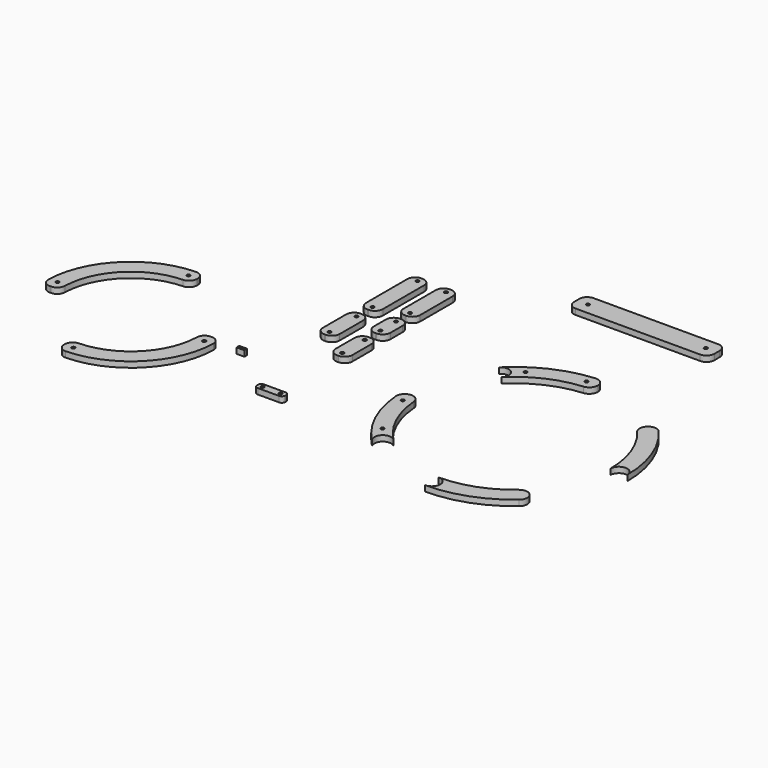
from build123d import *

# Parameters (mm, degrees)
F0_R     = 1.5
F1_DEPTH = 5.08
F0_W     = 7
F0_H     = 3
F0_W_2   = 5.08
F0_H_2   = 1.5
F0_W_3   = 12.5
F0_H_3   = 7
F0_W_4   = 15
F0_H_4   = 60
F0_H_5   = 40
F0_H_6   = 35
F0_H_7   = 27.5
F0_H_8   = 50
F0_W_5   = 125
F0_H_9   = 20
F2_R     = 7
F2_2_R   = 7
F2_3_R   = 7
F2_4_R   = 7
F2_5_R   = 7
F2_6_R   = 7
F2_7_R   = 7
F2_8_R   = 7
F3_R     = 3
F4_R     = 7.49999
F4_2_R   = 7.49999
F4_3_R   = 7.49999
F4_4_R   = 7.49999


# Not quite as in the source:
# - a fillet or chamfer is up to 0.001 mm smaller than in the source, because OpenCascade refuses the exact size
# - a feature names something its author has since deleted; it is built from what else it names


with BuildPart() as f1:
    # F0 (on Top) → F1 (new body)
    with BuildSketch(Plane.XY):
        with BuildLine():
            Line((-60.3335389302, 75.6855827492), (-60.3335389302, 90.7311393763))
            ThreePointArc((-60.3335389302, 90.7311393763), (-118.5826653378, 68.9457537369), (-140.3680509771, 10.6966273294))
            Line((-140.3680509771, 10.6966273294), (-125.32249435, 10.6966273294))
            ThreePointArc((-125.32249435, 10.6966273294), (-107.97606362, 58.3391520191), (-60.3335389302, 75.6855827492))
        make_face()
        with Locations((-133.0496567488, 18.6966273294)):
            Circle(F0_R, mode=Mode.SUBTRACT)
        with Locations((-68.3335389302, 83.4127451479)):
            Circle(F0_R, mode=Mode.SUBTRACT)
    extrude(amount=F1_DEPTH)

    # F2
    f2_edges = [f1.edges().sort_by_distance(p)[0] for p in [
        (-140.368051, 10.696627, 2.54),
        (-125.322494, 10.696627, 2.54),
        (-60.333539, 90.731139, 2.54),
        (-60.333539, 75.685583, 2.54),
    ]]
    fillet(f2_edges, radius=F2_R)


with BuildPart() as f1b:
    # F0 (on Top) → F1, piece 2 (new body)
    with BuildSketch(Plane.XY):
        with BuildLine():
            ThreePointArc((-70.7657745674, -58.9056490804), (-14.3940550828, -38.933443582), (9.4503432512, 15.9127451479))
            ThreePointArc((9.4503432512, 15.9127451479), (9.404928058, 18.5223842874), (9.2687374795, 21.1288629665))
            Line((9.2687374795, 21.1288629665), (-5.7768191475, 21.1288629665))
            ThreePointArc((-5.7768191475, 21.1288629665), (-5.6064742504, 18.5232761214), (-5.5496567488, 15.9127451479))
            ThreePointArc((-5.5496567488, 15.9127451479), (-25.0093500721, -28.3194098364), (-70.7657745674, -43.8600924533))
            Line((-70.7657745674, -43.8600924533), (-70.7657745674, -58.9056490804))
        make_face()
        with Locations((-62.7657745674, -51.5872548521)):
            Circle(F0_R, mode=Mode.SUBTRACT)
        with Locations((1.9503432512, 13.1288629665)):
            Circle(F0_R, mode=Mode.SUBTRACT)
    extrude(amount=F1_DEPTH)

    # F2#2
    f2_2_edges = [f1b.edges().sort_by_distance(p)[0] for p in [
        (-5.776819, 21.128863, 2.54),
        (9.268737, 21.128863, 2.54),
        (-70.765775, -43.860092, 2.54),
        (-70.765775, -58.905649, 2.54),
    ]]
    fillet(f2_2_edges, radius=F2_2_R)


with BuildPart() as f1c:
    # F0 (on Top) → F1, piece 3 (new body)
    with BuildSketch(Plane.XY):
        with Locations((29.0703890151, 21.1699748555)):
            Rectangle(F0_W, F0_H)
        with Locations((29.0703890151, 21.1699748555)):
            Rectangle(F0_W_2, F0_H_2, mode=Mode.SUBTRACT)
    extrude(amount=F1_DEPTH)


with BuildPart() as f1d:
    # F0 (on Top) → F1, piece 4 (new body)
    with BuildSketch(Plane.XY):
        with Locations((78.5480350256, -15.4045127481)):
            Rectangle(F0_W_3, F0_H_3)
        with Locations((76.7980350256, -15.4045127481)):
            Circle(F0_R, mode=Mode.SUBTRACT)
        with Locations((91.0480350256, -15.4045127481)):
            Rectangle(F0_W_3, F0_H_3)
        with Locations((92.7980350256, -15.4045127481)):
            Circle(F0_R, mode=Mode.SUBTRACT)
    extrude(amount=F1_DEPTH)

    # F3
    f3_edges = [f1d.edges().sort_by_distance(p)[0] for p in [
        (72.298035, -11.904513, 2.54),
        (72.298035, -18.904513, 2.54),
        (97.298035, -11.904513, 2.54),
        (97.298035, -18.904513, 2.54),
    ]]
    fillet(f3_edges, radius=F3_R)


with BuildPart() as f1e:
    # F0 (on Top) → F1, piece 5 (new body)
    with BuildSketch(Plane.XY):
        with BuildLine():
            Line((257.5643956661, 124.5856685936), (257.5643956661, 139.5856685936))
            ThreePointArc((257.5643956661, 139.5856685936), (219.2960524296, 131.9736218448), (186.8537175475, 110.2963467123))
            ThreePointArc((186.8537175475, 110.2963467123), (197.4603192653, 110.2963467123), (197.4603192653, 99.6897449945))
            ThreePointArc((197.4603192653, 99.6897449945), (225.0363039151, 118.1154288571), (257.5643956661, 124.5856685936))
        make_face()
        with Locations((205.6464472819, 116.1413779534)):
            Circle(F0_R, mode=Mode.SUBTRACT)
        with Locations((247.5643956661, 131.5435393824)):
            Circle(F0_R, mode=Mode.SUBTRACT)
    extrude(amount=F1_DEPTH)

    # F4 (radius 7.5 in the source; OpenCascade refuses exactly that, so slightly less here)
    f4_edges = [f1e.edges().sort_by_distance(p)[0] for p in [
        (257.564396, 139.585669, 2.54),
        (257.564396, 124.585669, 2.54),
    ]]
    fillet(f4_edges, radius=F4_R)


with BuildPart() as f1f:
    # F0 (on Top) → F1, piece 6 (new body)
    with BuildSketch(Plane.XY):
        with BuildLine():
            ThreePointArc((342.5643956661, 39.5856685936), (350.0643956661, 47.0856685936), (357.5643956661, 39.5856685936))
            ThreePointArc((357.5643956661, 39.5856685936), (349.9523489173, 77.8540118302), (328.2750737848, 110.2963467123))
            Line((328.2750737848, 110.2963467123), (317.668472067, 99.6897449945))
            ThreePointArc((317.668472067, 99.6897449945), (336.0941559296, 72.1137603447), (342.5643956661, 39.5856685936))
        make_face()
    extrude(amount=F1_DEPTH)

    # F4#2 (radius 7.5 in the source; OpenCascade refuses exactly that, so slightly less here)
    f4_2_edges = [f1f.edges().sort_by_distance(p)[0] for p in [
        (328.275074, 110.296347, 2.54),
        (317.668472, 99.689745, 2.54),
    ]]
    fillet(f4_2_edges, radius=F4_2_R)


with BuildPart() as f1g:
    # F0 (on Top) → F1, piece 7 (new body)
    with BuildSketch(Plane.XY):
        with BuildLine():
            ThreePointArc((157.5643956661, 39.5856685936), (165.176442415, 1.3173253571), (186.8537175475, -31.125009525))
            ThreePointArc((186.8537175475, -31.125009525), (186.8537175475, -20.5184078072), (197.4603192653, -20.5184078072))
            ThreePointArc((197.4603192653, -20.5184078072), (179.0346354027, 7.0575768426), (172.5643956661, 39.5856685936))
            Line((172.5643956661, 39.5856685936), (157.5643956661, 39.5856685936))
        make_face()
        with Locations((181.0086863064, -12.3322797906)):
            Circle(F0_R, mode=Mode.SUBTRACT)
        with Locations((165.6065248774, 29.5856685936)):
            Circle(F0_R, mode=Mode.SUBTRACT)
    extrude(amount=F1_DEPTH)

    # F4#4 (radius 7.5 in the source; OpenCascade refuses exactly that, so slightly less here)
    f4_4_edges = [f1g.edges().sort_by_distance(p)[0] for p in [
        (157.564396, 39.585669, 2.54),
        (172.564396, 39.585669, 2.54),
    ]]
    fillet(f4_4_edges, radius=F4_4_R)


with BuildPart() as f1h:
    # F0 (on Top) → F1, piece 8 (new body)
    with BuildSketch(Plane.XY):
        with BuildLine():
            ThreePointArc((257.5643956661, -60.4143314064), (295.8327389026, -52.8022846575), (328.2750737848, -31.125009525))
            Line((328.2750737848, -31.125009525), (317.668472067, -20.5184078072))
            ThreePointArc((317.668472067, -20.5184078072), (290.0924874172, -38.9440916698), (257.5643956661, -45.4143314064))
            ThreePointArc((257.5643956661, -45.4143314064), (265.0643956661, -52.9143314064), (257.5643956661, -60.4143314064))
        make_face()
    extrude(amount=F1_DEPTH)

    # F4#3 (radius 7.5 in the source; OpenCascade refuses exactly that, so slightly less here)
    f4_3_edges = [f1h.edges().sort_by_distance(p)[0] for p in [
        (317.668472, -20.518408, 2.54),
        (328.275074, -31.12501, 2.54),
    ]]
    fillet(f4_3_edges, radius=F4_3_R)


with BuildPart() as f1i:
    # F0 (on Top) → F1, piece 9 (new body)
    with BuildSketch(Plane.XY):
        with Locations((61.4713911712, 151.1703047156)):
            Rectangle(F0_W_4, F0_H_4)
        with Locations((61.4713911712, 126.1703047156)):
            Circle(F0_R, mode=Mode.SUBTRACT)
        with Locations((61.4713911712, 176.1703047156)):
            Circle(F0_R, mode=Mode.SUBTRACT)
    extrude(amount=F1_DEPTH)

    # F2#3
    f2_3_edges = [f1i.edges().sort_by_distance(p)[0] for p in [
        (68.971391, 181.170305, 2.54),
        (53.971391, 181.170305, 2.54),
        (53.971391, 121.170305, 2.54),
        (68.971391, 121.170305, 2.54),
    ]]
    fillet(f2_3_edges, radius=F2_3_R)


with BuildPart() as f1j:
    # F0 (on Top) → F1, piece 10 (new body)
    with BuildSketch(Plane.XY):
        with Locations((61.4713911712, 93.2305198908)):
            Rectangle(F0_W_4, F0_H_5)
        with Locations((61.4713911712, 78.2305198908)):
            Circle(F0_R, mode=Mode.SUBTRACT)
        with Locations((61.4713911712, 108.2305198908)):
            Circle(F0_R, mode=Mode.SUBTRACT)
    extrude(amount=F1_DEPTH)

    # F2#4
    f2_4_edges = [f1j.edges().sort_by_distance(p)[0] for p in [
        (53.971391, 113.23052, 2.54),
        (68.971391, 113.23052, 2.54),
        (68.971391, 73.23052, 2.54),
        (53.971391, 73.23052, 2.54),
    ]]
    fillet(f2_4_edges, radius=F2_4_R)


with BuildPart() as f1k:
    # F0 (on Top) → F1, piece 11 (new body)
    with BuildSketch(Plane.XY):
        with Locations((88.1428641081, 71.6127920151)):
            Rectangle(F0_W_4, F0_H_6)
        with Locations((88.1428641081, 59.1127920151)):
            Circle(F0_R, mode=Mode.SUBTRACT)
        with Locations((88.1428641081, 84.1127920151)):
            Circle(F0_R, mode=Mode.SUBTRACT)
    extrude(amount=F1_DEPTH)

    # F2#5
    f2_5_edges = [f1k.edges().sort_by_distance(p)[0] for p in [
        (95.642864, 54.112792, 2.54),
        (80.642864, 54.112792, 2.54),
        (80.642864, 89.112792, 2.54),
        (95.642864, 89.112792, 2.54),
    ]]
    fillet(f2_5_edges, radius=F2_5_R)


with BuildPart() as f1l:
    # F0 (on Top) → F1, piece 12 (new body)
    with BuildSketch(Plane.XY):
        with Locations((87.84070611, 110.5955246091)):
            Rectangle(F0_W_4, F0_H_7)
        with BuildLine():
            ThreePointArc((89.34070611, 101.8455246091), (86.7800459382, 100.7848644373), (87.84070611, 103.3455246091))
            ThreePointArc((87.84070611, 103.3455246091), (88.9013662818, 102.9061847809), (89.34070611, 101.8455246091))
        make_face(mode=Mode.SUBTRACT)
        with BuildLine():
            ThreePointArc((89.34070611, 119.3455246091), (88.9013662818, 118.2848644373), (87.84070611, 117.8455246091))
            ThreePointArc((87.84070611, 117.8455246091), (86.7800459382, 120.4061847809), (89.34070611, 119.3455246091))
        make_face(mode=Mode.SUBTRACT)
    extrude(amount=F1_DEPTH)

    # F2#6
    f2_6_edges = [f1l.edges().sort_by_distance(p)[0] for p in [
        (80.340706, 124.345525, 2.54),
        (95.340706, 124.345525, 2.54),
        (95.340706, 96.845525, 2.54),
        (80.340706, 96.845525, 2.54),
    ]]
    fillet(f2_6_edges, radius=F2_6_R)


with BuildPart() as f1m:
    # F0 (on Top) → F1, piece 13 (new body)
    with BuildSketch(Plane.XY):
        with Locations((87.326824367, 155.552560091)):
            Rectangle(F0_W_4, F0_H_8)
        with Locations((87.326824367, 135.552560091)):
            Circle(F0_R, mode=Mode.SUBTRACT)
        with Locations((87.326824367, 175.552560091)):
            Circle(F0_R, mode=Mode.SUBTRACT)
    extrude(amount=F1_DEPTH)

    # F2#7
    f2_7_edges = [f1m.edges().sort_by_distance(p)[0] for p in [
        (94.826824, 130.55256, 2.54),
        (79.826824, 130.55256, 2.54),
        (79.826824, 180.55256, 2.54),
        (94.826824, 180.55256, 2.54),
    ]]
    fillet(f2_7_edges, radius=F2_7_R)


with BuildPart() as f1n:
    # F0 (on Top) → F1, piece 14 (new body)
    with BuildSketch(Plane.XY):
        with Locations((228.5025268793, 222.6880139112)):
            Rectangle(F0_W_5, F0_H_9)
        with Locations((176.0025268793, 222.6880139112)):
            Circle(F0_R, mode=Mode.SUBTRACT)
        with Locations((281.0025268793, 222.6880139112)):
            Circle(F0_R, mode=Mode.SUBTRACT)
    extrude(amount=F1_DEPTH)

    # F2#8
    f2_8_edges = [f1n.edges().sort_by_distance(p)[0] for p in [
        (166.002527, 232.688014, 2.54),
        (166.002527, 212.688014, 2.54),
        (291.002527, 232.688014, 2.54),
        (291.002527, 212.688014, 2.54),
    ]]
    fillet(f2_8_edges, radius=F2_8_R)


solid = Compound([f1.part, f1b.part, f1c.part, f1d.part, f1e.part, f1f.part, f1g.part, f1h.part, f1i.part, f1j.part, f1k.part, f1l.part, f1m.part, f1n.part])
